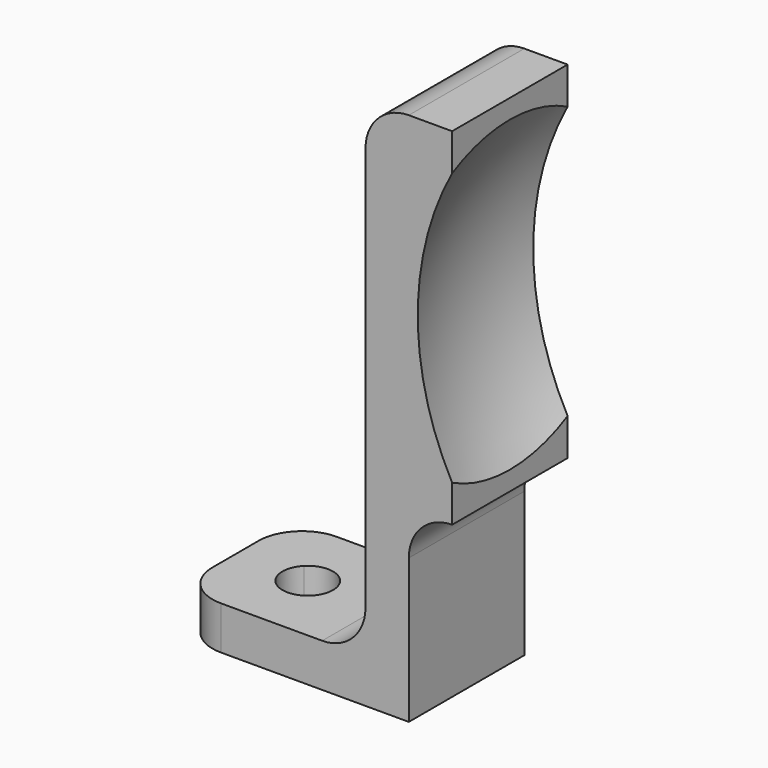
from build123d import *

# Parameters (mm, degrees)
F1_W          = 3
F1_H          = 12
F2_DEPTH      = 5
F2_DEPTH_BACK = 5
F4_R          = 3
F5_R          = 2.99999
F7_DEPTH      = 25
F8_R          = 3


# Not quite as in the source:
# - a fillet or chamfer is up to 0.001 mm smaller than in the source, because OpenCascade refuses the exact size


with BuildPart() as f2:
    # F1 (on Front) → F2 (new body, two sides)
    with BuildSketch(Plane.XZ) as f2_sk:
        with Locations((-19, -6)):
            Rectangle(F1_W, F1_H)
        Polygon((-20.5, 0), (-17.5, 0), (-17.5, 12), (-23.5, 12), (-23.5, -22), (-36.5, -22), (-36.5, -25), (-20.5, -25), (-20.5, -12), align=None)
    extrude(amount=F2_DEPTH)
    extrude(f2_sk.sketch, amount=-F2_DEPTH_BACK)

    # F0 (on Front) → F3 (revolve, cut)
    with BuildSketch(Plane.XZ):
        with BuildLine():
            Line((0, -20.5), (0, 20.5))
            ThreePointArc((0, 20.5), (-20.5, 0), (0, -20.5))
        make_face()
    revolve(axis=Axis((0, 0, 0), (0, 0, 1)), mode=Mode.SUBTRACT)

    # F4
    f4_edges = [f2.edges().sort_by_distance(p)[0] for p in [
        (-23.5, 0, 12),
        (-23.5, 0, -22),
    ]]
    fillet(f4_edges, radius=F4_R)

    # F5 (radius 3 in the source; OpenCascade refuses exactly that, so slightly less here)
    f5_edges = [f2.edges().sort_by_distance(p)[0] for p in [
        (-20.5, 0, -12),
    ]]
    fillet(f5_edges, radius=F5_R)

    # F6 (on face) → F7 (cut)
    with BuildSketch(Plane.XY.offset(-22)):
        with BuildLine():
            ThreePointArc((-29.75, 0), (-30.8303039934, 1.6167891819), (-32.7374368671, 1.2374368671))
            Line((-32.7374368671, 1.2374368671), (-30.2625631329, -1.2374368671))
            ThreePointArc((-30.2625631329, -1.2374368671), (-29.8832108181, -0.6696960066), (-29.75, 0))
        make_face()
        with BuildLine():
            Line((-30.2625631329, -1.2374368671), (-32.7374368671, 1.2374368671))
            ThreePointArc((-32.7374368671, 1.2374368671), (-32.7374368671, -1.2374368671), (-30.2625631329, -1.2374368671))
        make_face()
    extrude(amount=-F7_DEPTH, mode=Mode.SUBTRACT)

    # F8
    f8_edges = [f2.edges().sort_by_distance(p)[0] for p in [
        (-36.5, -5, -23.5),
        (-36.5, 5, -23.5),
    ]]
    fillet(f8_edges, radius=F8_R)


solid = f2.part
